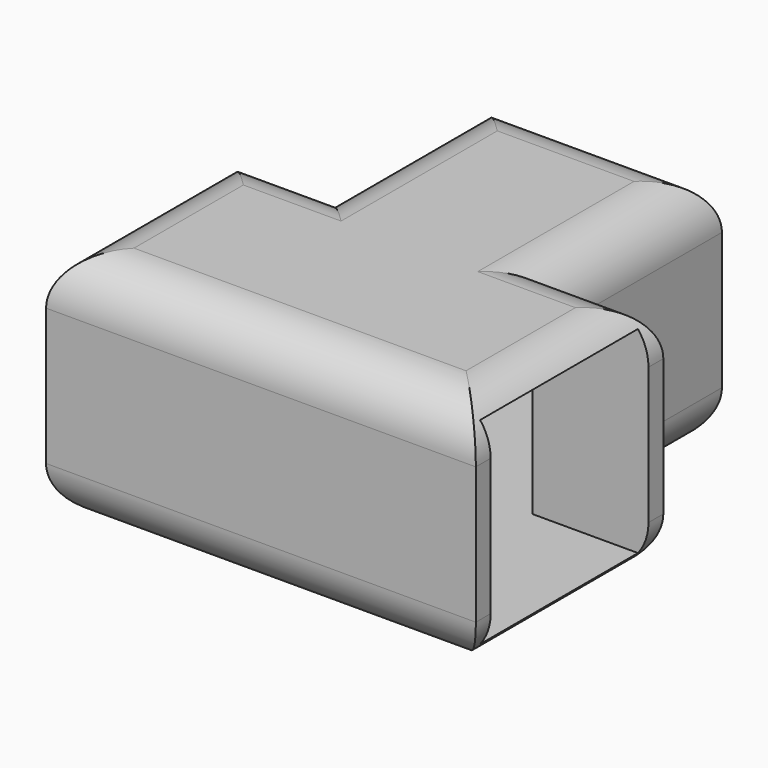
from build123d import *

# Parameters (mm, degrees)
F0_W          = 10
F0_H          = 24
F0_W_2        = 24
F0_H_2        = 20
F1_DEPTH      = 24
F2_T          = -1.9
F3_T1_DEPTH   = 44
F3_T3_DEPTH   = 24
F3_T5_DEPTH   = 10
F3_T7_DEPTH   = 20
F3_T9_DEPTH   = 24
F3_T11_DEPTH  = 10
F3_T17_DEPTH  = 56.5
F3_T21_DEPTH  = 36.5
F3_T28_DEPTH  = 56.5
F3_T32_DEPTH  = 36.5
F3_T39_DEPTH  = 22.5
F3_T43_DEPTH  = 36.5
F3_T50_DEPTH  = 22.5
F3_T54_DEPTH  = 32.5
F3_T61_DEPTH  = 32.5
F3_T65_DEPTH  = 36.5
F3_T72_DEPTH  = 32.5
F3_T76_DEPTH  = 36.5
F3_T83_DEPTH  = 32.5
F3_T87_DEPTH  = 22.5
F3_T94_DEPTH  = 22.5
F3_T98_DEPTH  = 36.5
F3_T105_DEPTH = 56.5
F3_T109_DEPTH = 36.5
F3_T116_DEPTH = 56.5
F3_T120_DEPTH = 36.5
F3_T127_DEPTH = 36.5
F3_T131_DEPTH = 22.5
F3_T138_DEPTH = 22.5
F3_T142_DEPTH = 32.5
F3_T149_DEPTH = 32.5
F3_T153_DEPTH = 36.5
F3_T160_DEPTH = 36.5
F3_T164_DEPTH = 32.5
F3_T171_DEPTH = 32.5
F3_T175_DEPTH = 22.5
F3_T182_DEPTH = 22.5
F3_T186_DEPTH = 36.5


# Not quite as in the source:
# - a fillet or chamfer that OpenCascade refuses, or shapes differently, is made with other operations: its cross-section is extruded or revolved along the edge and cut away or added


with BuildPart() as f1:
    # F0 (on Top) → F1 (new body)
    with BuildSketch(Plane.XY):
        with Locations((-16.1171973497, 12)):
            Rectangle(F0_W, F0_H)
        with Locations((0.8828026503, 12)):
            Rectangle(F0_W_2, F0_H)
        with Locations((17.8828026503, 12)):
            Rectangle(F0_W, F0_H)
        with Locations((0.8828026503, 34)):
            Rectangle(F0_W_2, F0_H_2)
    extrude(amount=F1_DEPTH)

    # F2
    f2_openings = [f1.faces().sort_by_distance(p)[0] for p in [
        (-21.117197, 12, 12),
        (22.882803, 12, 12),
        (0.882803, 44, 12),
    ]]
    offset(amount=F2_T, openings=f2_openings, kind=Kind.INTERSECTION)

    # F3: fillet of radius 5 on 16 edges, made by hand

    # F3_s2 → F3_t1 (cut)
    with BuildSketch(Plane.YZ.offset(-21.1171973497)):
        with BuildLine():
            ThreePointArc((0, 19), (1.4644660941, 22.5355339059), (5, 24))
            Line((5, 24), (5, 24.1))
            Line((5, 24.1), (-0.1, 24.1))
            Line((-0.1, 24.1), (-0.1, 19))
            Line((-0.1, 19), (0, 19))
        make_face()
        with BuildLine():
            ThreePointArc((0, 5), (1.4644660941, 1.4644660941), (5, 0))
            Line((5, 0), (5, -0.1))
            Line((5, -0.1), (-0.1, -0.1))
            Line((-0.1, -0.1), (-0.1, 5))
            Line((-0.1, 5), (0, 5))
        make_face()
    extrude(amount=F3_T1_DEPTH, mode=Mode.SUBTRACT)

    # F3_s4 → F3_t3 (cut)
    with BuildSketch(Plane.XZ.offset(-24)):
        with BuildLine():
            ThreePointArc((17.8828026503, 24), (21.4183365563, 22.5355339059), (22.8828026503, 19))
            Line((22.8828026503, 19), (22.9828026503, 19))
            Line((22.9828026503, 19), (22.9828026503, 24.1))
            Line((22.9828026503, 24.1), (17.8828026503, 24.1))
            Line((17.8828026503, 24.1), (17.8828026503, 24))
        make_face()
        with BuildLine():
            ThreePointArc((-16.1171973497, 24), (-19.6527312556, 22.5355339059), (-21.1171973497, 19))
            Line((-21.1171973497, 19), (-21.2171973497, 19))
            Line((-21.2171973497, 19), (-21.2171973497, 24.1))
            Line((-21.2171973497, 24.1), (-16.1171973497, 24.1))
            Line((-16.1171973497, 24.1), (-16.1171973497, 24))
        make_face()
        with BuildLine():
            ThreePointArc((17.8828026503, 0), (21.4183365563, 1.4644660941), (22.8828026503, 5))
            Line((22.8828026503, 5), (22.9828026503, 5))
            Line((22.9828026503, 5), (22.9828026503, -0.1))
            Line((22.9828026503, -0.1), (17.8828026503, -0.1))
            Line((17.8828026503, -0.1), (17.8828026503, 0))
        make_face()
        with BuildLine():
            ThreePointArc((-16.1171973497, 0), (-19.6527312556, 1.4644660941), (-21.1171973497, 5))
            Line((-21.1171973497, 5), (-21.2171973497, 5))
            Line((-21.2171973497, 5), (-21.2171973497, -0.1))
            Line((-21.2171973497, -0.1), (-16.1171973497, -0.1))
            Line((-16.1171973497, -0.1), (-16.1171973497, 0))
        make_face()
    extrude(amount=F3_T3_DEPTH, mode=Mode.SUBTRACT)

    # F3_s6 → F3_t5 (cut)
    with BuildSketch(Plane.YZ.offset(12.8828026503)):
        with BuildLine():
            ThreePointArc((24, 19), (22.5355339059, 22.5355339059), (19, 24))
            Line((19, 24), (19, 24.1))
            Line((19, 24.1), (24.1, 24.1))
            Line((24.1, 24.1), (24.1, 19))
            Line((24.1, 19), (24, 19))
        make_face()
        with BuildLine():
            ThreePointArc((19, 0), (22.5355339059, 1.4644660941), (24, 5))
            Line((24, 5), (24.1, 5))
            Line((24.1, 5), (24.1, -0.1))
            Line((24.1, -0.1), (19, -0.1))
            Line((19, -0.1), (19, 0))
        make_face()
    extrude(amount=F3_T5_DEPTH, mode=Mode.SUBTRACT)

    # F3_s8 → F3_t7 (cut)
    with BuildSketch(Plane.XZ.offset(-44)):
        with BuildLine():
            ThreePointArc((12.8828026503, 19), (11.4183365563, 22.5355339059), (7.8828026503, 24))
            Line((7.8828026503, 24), (7.8828026503, 24.1))
            Line((7.8828026503, 24.1), (12.9828026503, 24.1))
            Line((12.9828026503, 24.1), (12.9828026503, 19))
            Line((12.9828026503, 19), (12.8828026503, 19))
        make_face()
        with BuildLine():
            ThreePointArc((-11.1171973497, 19), (-9.6527312556, 22.5355339059), (-6.1171973497, 24))
            Line((-6.1171973497, 24), (-6.1171973497, 24.1))
            Line((-6.1171973497, 24.1), (-11.2171973497, 24.1))
            Line((-11.2171973497, 24.1), (-11.2171973497, 19))
            Line((-11.2171973497, 19), (-11.1171973497, 19))
        make_face()
        with BuildLine():
            ThreePointArc((7.8828026503, 0), (11.4183365563, 1.4644660941), (12.8828026503, 5))
            Line((12.8828026503, 5), (12.9828026503, 5))
            Line((12.9828026503, 5), (12.9828026503, -0.1))
            Line((12.9828026503, -0.1), (7.8828026503, -0.1))
            Line((7.8828026503, -0.1), (7.8828026503, 0))
        make_face()
        with BuildLine():
            ThreePointArc((-6.1171973497, 0), (-9.6527312556, 1.4644660941), (-11.1171973497, 5))
            Line((-11.1171973497, 5), (-11.2171973497, 5))
            Line((-11.2171973497, 5), (-11.2171973497, -0.1))
            Line((-11.2171973497, -0.1), (-6.1171973497, -0.1))
            Line((-6.1171973497, -0.1), (-6.1171973497, 0))
        make_face()
    extrude(amount=F3_T7_DEPTH, mode=Mode.SUBTRACT)

    # F3_s10 → F3_t9 (cut)
    with BuildSketch(Plane.YZ.offset(-11.1171973497)):
        with BuildLine():
            ThreePointArc((39, 24), (42.5355339059, 22.5355339059), (44, 19))
            Line((44, 19), (44.1, 19))
            Line((44.1, 19), (44.1, 24.1))
            Line((44.1, 24.1), (39, 24.1))
            Line((39, 24.1), (39, 24))
        make_face()
        with BuildLine():
            ThreePointArc((39, 0), (42.5355339059, 1.4644660941), (44, 5))
            Line((44, 5), (44.1, 5))
            Line((44.1, 5), (44.1, -0.1))
            Line((44.1, -0.1), (39, -0.1))
            Line((39, -0.1), (39, 0))
        make_face()
    extrude(amount=F3_T9_DEPTH, mode=Mode.SUBTRACT)

    # F3_s12 → F3_t11 (cut)
    with BuildSketch(Plane.YZ.offset(-21.1171973497)):
        with BuildLine():
            ThreePointArc((24, 19), (22.5355339059, 22.5355339059), (19, 24))
            Line((19, 24), (19, 24.1))
            Line((19, 24.1), (24.1, 24.1))
            Line((24.1, 24.1), (24.1, 19))
            Line((24.1, 19), (24, 19))
        make_face()
        with BuildLine():
            ThreePointArc((19, 0), (22.5355339059, 1.4644660941), (24, 5))
            Line((24, 5), (24.1, 5))
            Line((24.1, 5), (24.1, -0.1))
            Line((24.1, -0.1), (19, -0.1))
            Line((19, -0.1), (19, 0))
        make_face()
    extrude(amount=F3_T11_DEPTH, mode=Mode.SUBTRACT)


with BuildPart() as f3_tool15:
    # F3_s16 → F3_t17 (new body)
    with BuildSketch(Plane.YZ.offset(-33.6171973497)):
        with BuildLine():
            ThreePointArc((0, 19), (1.4644660941, 22.5355339059), (5, 24))
            Line((5, 24), (5, 24.1))
            Line((5, 24.1), (-0.1, 24.1))
            Line((-0.1, 24.1), (-0.1, 19))
            Line((-0.1, 19), (0, 19))
        make_face()
    extrude(amount=F3_T17_DEPTH)

    split(bisect_by=Plane.YZ.offset(-21.1171973497), keep=Keep.BOTTOM)


with BuildPart() as f3_tool19:
    # F3_s20 → F3_t21 (new body)
    with BuildSketch(Plane.XZ.offset(-24)):
        with BuildLine():
            ThreePointArc((-16.1171973497, 24), (-19.6527312556, 22.5355339059), (-21.1171973497, 19))
            Line((-21.1171973497, 19), (-21.2171973497, 19))
            Line((-21.2171973497, 19), (-21.2171973497, 24.1))
            Line((-21.2171973497, 24.1), (-16.1171973497, 24.1))
            Line((-16.1171973497, 24.1), (-16.1171973497, 24))
        make_face()
    extrude(amount=F3_T21_DEPTH)

    split(bisect_by=Plane.XZ, keep=Keep.TOP)


with BuildPart() as f3_tool15_1:
    add(f3_tool15.part)

    # F3_t23: intersect F3_tool19
    add(f3_tool19.part, mode=Mode.INTERSECT)


with BuildPart() as f1_1:
    add(f1.part)

    # F3_t13: cut F3_tool15
    add(f3_tool15_1.part, mode=Mode.SUBTRACT)


with BuildPart() as f3_tool26:
    # F3_s27 → F3_t28 (new body)
    with BuildSketch(Plane.YZ.offset(-21.1171973497)):
        with BuildLine():
            ThreePointArc((0, 19), (1.4644660941, 22.5355339059), (5, 24))
            Line((5, 24), (5, 24.1))
            Line((5, 24.1), (-0.1, 24.1))
            Line((-0.1, 24.1), (-0.1, 19))
            Line((-0.1, 19), (0, 19))
        make_face()
    extrude(amount=F3_T28_DEPTH)

    split(bisect_by=Plane.YZ.offset(22.8828026503), keep=Keep.TOP)


with BuildPart() as f3_tool30:
    # F3_s31 → F3_t32 (new body)
    with BuildSketch(Plane.XZ.offset(12.5)):
        with BuildLine():
            ThreePointArc((17.8828026503, 24), (21.4183365563, 22.5355339059), (22.8828026503, 19))
            Line((22.8828026503, 19), (22.9828026503, 19))
            Line((22.9828026503, 19), (22.9828026503, 24.1))
            Line((22.9828026503, 24.1), (17.8828026503, 24.1))
            Line((17.8828026503, 24.1), (17.8828026503, 24))
        make_face()
    extrude(amount=-F3_T32_DEPTH)

    split(bisect_by=Plane.XZ, keep=Keep.TOP)


with BuildPart() as f3_tool26_1:
    add(f3_tool26.part)

    # F3_t34: intersect F3_tool30
    add(f3_tool30.part, mode=Mode.INTERSECT)


with BuildPart() as f1_2:
    add(f1_1.part)

    # F3_t24: cut F3_tool26
    add(f3_tool26_1.part, mode=Mode.SUBTRACT)


with BuildPart() as f3_tool37:
    # F3_s38 → F3_t39 (new body)
    with BuildSketch(Plane.YZ.offset(35.3828026503)):
        with BuildLine():
            ThreePointArc((24, 19), (22.5355339059, 22.5355339059), (19, 24))
            Line((19, 24), (19, 24.1))
            Line((19, 24.1), (24.1, 24.1))
            Line((24.1, 24.1), (24.1, 19))
            Line((24.1, 19), (24, 19))
        make_face()
    extrude(amount=-F3_T39_DEPTH)

    split(bisect_by=Plane.YZ.offset(22.8828026503), keep=Keep.TOP)


with BuildPart() as f3_tool41:
    # F3_s42 → F3_t43 (new body)
    with BuildSketch(Plane.XZ):
        with BuildLine():
            ThreePointArc((17.8828026503, 24), (21.4183365563, 22.5355339059), (22.8828026503, 19))
            Line((22.8828026503, 19), (22.9828026503, 19))
            Line((22.9828026503, 19), (22.9828026503, 24.1))
            Line((22.9828026503, 24.1), (17.8828026503, 24.1))
            Line((17.8828026503, 24.1), (17.8828026503, 24))
        make_face()
    extrude(amount=-F3_T43_DEPTH)

    split(bisect_by=Plane.XZ.offset(-24), keep=Keep.BOTTOM)


with BuildPart() as f3_tool37_1:
    add(f3_tool37.part)

    # F3_t45: intersect F3_tool41
    add(f3_tool41.part, mode=Mode.INTERSECT)


with BuildPart() as f1_3:
    add(f1_2.part)

    # F3_t35: cut F3_tool37
    add(f3_tool37_1.part, mode=Mode.SUBTRACT)


with BuildPart() as f3_tool48:
    # F3_s49 → F3_t50 (new body)
    with BuildSketch(Plane.YZ.offset(22.8828026503)):
        with BuildLine():
            ThreePointArc((24, 19), (22.5355339059, 22.5355339059), (19, 24))
            Line((19, 24), (19, 24.1))
            Line((19, 24.1), (24.1, 24.1))
            Line((24.1, 24.1), (24.1, 19))
            Line((24.1, 19), (24, 19))
        make_face()
    extrude(amount=-F3_T50_DEPTH)

    split(bisect_by=Plane.YZ.offset(12.8828026503), keep=Keep.BOTTOM)


with BuildPart() as f3_tool52:
    # F3_s53 → F3_t54 (new body)
    with BuildSketch(Plane.XZ.offset(-11.5)):
        with BuildLine():
            ThreePointArc((12.8828026503, 19), (11.4183365563, 22.5355339059), (7.8828026503, 24))
            Line((7.8828026503, 24), (7.8828026503, 24.1))
            Line((7.8828026503, 24.1), (12.9828026503, 24.1))
            Line((12.9828026503, 24.1), (12.9828026503, 19))
            Line((12.9828026503, 19), (12.8828026503, 19))
        make_face()
    extrude(amount=-F3_T54_DEPTH)

    split(bisect_by=Plane.XZ.offset(-24), keep=Keep.TOP)


with BuildPart() as f3_tool48_1:
    add(f3_tool48.part)

    # F3_t56: intersect F3_tool52
    add(f3_tool52.part, mode=Mode.INTERSECT)


with BuildPart() as f1_4:
    add(f1_3.part)

    # F3_t46: cut F3_tool48
    add(f3_tool48_1.part, mode=Mode.SUBTRACT)


with BuildPart() as f3_tool59:
    # F3_s60 → F3_t61 (new body)
    with BuildSketch(Plane.XZ.offset(-24)):
        with BuildLine():
            ThreePointArc((12.8828026503, 19), (11.4183365563, 22.5355339059), (7.8828026503, 24))
            Line((7.8828026503, 24), (7.8828026503, 24.1))
            Line((7.8828026503, 24.1), (12.9828026503, 24.1))
            Line((12.9828026503, 24.1), (12.9828026503, 19))
            Line((12.9828026503, 19), (12.8828026503, 19))
        make_face()
    extrude(amount=-F3_T61_DEPTH)

    split(bisect_by=Plane.XZ.offset(-44), keep=Keep.BOTTOM)


with BuildPart() as f3_tool63:
    # F3_s64 → F3_t65 (new body)
    with BuildSketch(Plane.YZ.offset(25.3828026503)):
        with BuildLine():
            ThreePointArc((39, 24), (42.5355339059, 22.5355339059), (44, 19))
            Line((44, 19), (44.1, 19))
            Line((44.1, 19), (44.1, 24.1))
            Line((44.1, 24.1), (39, 24.1))
            Line((39, 24.1), (39, 24))
        make_face()
    extrude(amount=-F3_T65_DEPTH)

    split(bisect_by=Plane.YZ.offset(12.8828026503), keep=Keep.TOP)


with BuildPart() as f3_tool59_1:
    add(f3_tool59.part)

    # F3_t67: intersect F3_tool63
    add(f3_tool63.part, mode=Mode.INTERSECT)


with BuildPart() as f1_5:
    add(f1_4.part)

    # F3_t57: cut F3_tool59
    add(f3_tool59_1.part, mode=Mode.SUBTRACT)


with BuildPart() as f3_tool70:
    # F3_s71 → F3_t72 (new body)
    with BuildSketch(Plane.XZ.offset(-56.5)):
        with BuildLine():
            ThreePointArc((-11.1171973497, 19), (-9.6527312556, 22.5355339059), (-6.1171973497, 24))
            Line((-6.1171973497, 24), (-6.1171973497, 24.1))
            Line((-6.1171973497, 24.1), (-11.2171973497, 24.1))
            Line((-11.2171973497, 24.1), (-11.2171973497, 19))
            Line((-11.2171973497, 19), (-11.1171973497, 19))
        make_face()
    extrude(amount=F3_T72_DEPTH)

    split(bisect_by=Plane.XZ.offset(-44), keep=Keep.BOTTOM)


with BuildPart() as f3_tool74:
    # F3_s75 → F3_t76 (new body)
    with BuildSketch(Plane.YZ.offset(12.8828026503)):
        with BuildLine():
            ThreePointArc((39, 24), (42.5355339059, 22.5355339059), (44, 19))
            Line((44, 19), (44.1, 19))
            Line((44.1, 19), (44.1, 24.1))
            Line((44.1, 24.1), (39, 24.1))
            Line((39, 24.1), (39, 24))
        make_face()
    extrude(amount=-F3_T76_DEPTH)

    split(bisect_by=Plane.YZ.offset(-11.1171973497), keep=Keep.BOTTOM)


with BuildPart() as f3_tool70_1:
    add(f3_tool70.part)

    # F3_t78: intersect F3_tool74
    add(f3_tool74.part, mode=Mode.INTERSECT)


with BuildPart() as f1_6:
    add(f1_5.part)

    # F3_t68: cut F3_tool70
    add(f3_tool70_1.part, mode=Mode.SUBTRACT)


with BuildPart() as f3_tool81:
    # F3_s82 → F3_t83 (new body)
    with BuildSketch(Plane.XZ.offset(-44)):
        with BuildLine():
            ThreePointArc((-11.1171973497, 19), (-9.6527312556, 22.5355339059), (-6.1171973497, 24))
            Line((-6.1171973497, 24), (-6.1171973497, 24.1))
            Line((-6.1171973497, 24.1), (-11.2171973497, 24.1))
            Line((-11.2171973497, 24.1), (-11.2171973497, 19))
            Line((-11.2171973497, 19), (-11.1171973497, 19))
        make_face()
    extrude(amount=F3_T83_DEPTH)

    split(bisect_by=Plane.XZ.offset(-24), keep=Keep.TOP)


with BuildPart() as f3_tool85:
    # F3_s86 → F3_t87 (new body)
    with BuildSketch(Plane.YZ.offset(1.3828026503)):
        with BuildLine():
            ThreePointArc((24, 19), (22.5355339059, 22.5355339059), (19, 24))
            Line((19, 24), (19, 24.1))
            Line((19, 24.1), (24.1, 24.1))
            Line((24.1, 24.1), (24.1, 19))
            Line((24.1, 19), (24, 19))
        make_face()
    extrude(amount=-F3_T87_DEPTH)

    split(bisect_by=Plane.YZ.offset(-11.1171973497), keep=Keep.TOP)


with BuildPart() as f3_tool81_1:
    add(f3_tool81.part)

    # F3_t89: intersect F3_tool85
    add(f3_tool85.part, mode=Mode.INTERSECT)


with BuildPart() as f1_7:
    add(f1_6.part)

    # F3_t79: cut F3_tool81
    add(f3_tool81_1.part, mode=Mode.SUBTRACT)


with BuildPart() as f3_tool92:
    # F3_s93 → F3_t94 (new body)
    with BuildSketch(Plane.YZ.offset(-11.1171973497)):
        with BuildLine():
            ThreePointArc((24, 19), (22.5355339059, 22.5355339059), (19, 24))
            Line((19, 24), (19, 24.1))
            Line((19, 24.1), (24.1, 24.1))
            Line((24.1, 24.1), (24.1, 19))
            Line((24.1, 19), (24, 19))
        make_face()
    extrude(amount=-F3_T94_DEPTH)

    split(bisect_by=Plane.YZ.offset(-21.1171973497), keep=Keep.BOTTOM)


with BuildPart() as f3_tool96:
    # F3_s97 → F3_t98 (new body)
    with BuildSketch(Plane.XZ.offset(-36.5)):
        with BuildLine():
            ThreePointArc((-16.1171973497, 24), (-19.6527312556, 22.5355339059), (-21.1171973497, 19))
            Line((-21.1171973497, 19), (-21.2171973497, 19))
            Line((-21.2171973497, 19), (-21.2171973497, 24.1))
            Line((-21.2171973497, 24.1), (-16.1171973497, 24.1))
            Line((-16.1171973497, 24.1), (-16.1171973497, 24))
        make_face()
    extrude(amount=F3_T98_DEPTH)

    split(bisect_by=Plane.XZ.offset(-24), keep=Keep.BOTTOM)


with BuildPart() as f3_tool92_1:
    add(f3_tool92.part)

    # F3_t100: intersect F3_tool96
    add(f3_tool96.part, mode=Mode.INTERSECT)


with BuildPart() as f1_8:
    add(f1_7.part)

    # F3_t90: cut F3_tool92
    add(f3_tool92_1.part, mode=Mode.SUBTRACT)


with BuildPart() as f3_tool103:
    # F3_s104 → F3_t105 (new body)
    with BuildSketch(Plane.YZ.offset(-33.6171973497)):
        with BuildLine():
            ThreePointArc((0, 5), (1.4644660941, 1.4644660941), (5, 0))
            Line((5, 0), (5, -0.1))
            Line((5, -0.1), (-0.1, -0.1))
            Line((-0.1, -0.1), (-0.1, 5))
            Line((-0.1, 5), (0, 5))
        make_face()
    extrude(amount=F3_T105_DEPTH)

    split(bisect_by=Plane.YZ.offset(-21.1171973497), keep=Keep.BOTTOM)


with BuildPart() as f3_tool107:
    # F3_s108 → F3_t109 (new body)
    with BuildSketch(Plane.XZ.offset(-24)):
        with BuildLine():
            ThreePointArc((-16.1171973497, 0), (-19.6527312556, 1.4644660941), (-21.1171973497, 5))
            Line((-21.1171973497, 5), (-21.2171973497, 5))
            Line((-21.2171973497, 5), (-21.2171973497, -0.1))
            Line((-21.2171973497, -0.1), (-16.1171973497, -0.1))
            Line((-16.1171973497, -0.1), (-16.1171973497, 0))
        make_face()
    extrude(amount=F3_T109_DEPTH)

    split(bisect_by=Plane.XZ, keep=Keep.TOP)


with BuildPart() as f3_tool103_1:
    add(f3_tool103.part)

    # F3_t111: intersect F3_tool107
    add(f3_tool107.part, mode=Mode.INTERSECT)


with BuildPart() as f1_9:
    add(f1_8.part)

    # F3_t101: cut F3_tool103
    add(f3_tool103_1.part, mode=Mode.SUBTRACT)


with BuildPart() as f3_tool114:
    # F3_s115 → F3_t116 (new body)
    with BuildSketch(Plane.YZ.offset(-21.1171973497)):
        with BuildLine():
            ThreePointArc((0, 5), (1.4644660941, 1.4644660941), (5, 0))
            Line((5, 0), (5, -0.1))
            Line((5, -0.1), (-0.1, -0.1))
            Line((-0.1, -0.1), (-0.1, 5))
            Line((-0.1, 5), (0, 5))
        make_face()
    extrude(amount=F3_T116_DEPTH)

    split(bisect_by=Plane.YZ.offset(22.8828026503), keep=Keep.TOP)


with BuildPart() as f3_tool118:
    # F3_s119 → F3_t120 (new body)
    with BuildSketch(Plane.XZ.offset(12.5)):
        with BuildLine():
            ThreePointArc((17.8828026503, 0), (21.4183365563, 1.4644660941), (22.8828026503, 5))
            Line((22.8828026503, 5), (22.9828026503, 5))
            Line((22.9828026503, 5), (22.9828026503, -0.1))
            Line((22.9828026503, -0.1), (17.8828026503, -0.1))
            Line((17.8828026503, -0.1), (17.8828026503, 0))
        make_face()
    extrude(amount=-F3_T120_DEPTH)

    split(bisect_by=Plane.XZ, keep=Keep.TOP)


with BuildPart() as f3_tool114_1:
    add(f3_tool114.part)

    # F3_t122: intersect F3_tool118
    add(f3_tool118.part, mode=Mode.INTERSECT)


with BuildPart() as f1_10:
    add(f1_9.part)

    # F3_t112: cut F3_tool114
    add(f3_tool114_1.part, mode=Mode.SUBTRACT)


with BuildPart() as f3_tool125:
    # F3_s126 → F3_t127 (new body)
    with BuildSketch(Plane.XZ):
        with BuildLine():
            ThreePointArc((17.8828026503, 0), (21.4183365563, 1.4644660941), (22.8828026503, 5))
            Line((22.8828026503, 5), (22.9828026503, 5))
            Line((22.9828026503, 5), (22.9828026503, -0.1))
            Line((22.9828026503, -0.1), (17.8828026503, -0.1))
            Line((17.8828026503, -0.1), (17.8828026503, 0))
        make_face()
    extrude(amount=-F3_T127_DEPTH)

    split(bisect_by=Plane.XZ.offset(-24), keep=Keep.BOTTOM)


with BuildPart() as f3_tool129:
    # F3_s130 → F3_t131 (new body)
    with BuildSketch(Plane.YZ.offset(35.3828026503)):
        with BuildLine():
            ThreePointArc((19, 0), (22.5355339059, 1.4644660941), (24, 5))
            Line((24, 5), (24.1, 5))
            Line((24.1, 5), (24.1, -0.1))
            Line((24.1, -0.1), (19, -0.1))
            Line((19, -0.1), (19, 0))
        make_face()
    extrude(amount=-F3_T131_DEPTH)

    split(bisect_by=Plane.YZ.offset(22.8828026503), keep=Keep.TOP)


with BuildPart() as f3_tool125_1:
    add(f3_tool125.part)

    # F3_t133: intersect F3_tool129
    add(f3_tool129.part, mode=Mode.INTERSECT)


with BuildPart() as f1_11:
    add(f1_10.part)

    # F3_t123: cut F3_tool125
    add(f3_tool125_1.part, mode=Mode.SUBTRACT)


with BuildPart() as f3_tool136:
    # F3_s137 → F3_t138 (new body)
    with BuildSketch(Plane.YZ.offset(22.8828026503)):
        with BuildLine():
            ThreePointArc((19, 0), (22.5355339059, 1.4644660941), (24, 5))
            Line((24, 5), (24.1, 5))
            Line((24.1, 5), (24.1, -0.1))
            Line((24.1, -0.1), (19, -0.1))
            Line((19, -0.1), (19, 0))
        make_face()
    extrude(amount=-F3_T138_DEPTH)

    split(bisect_by=Plane.YZ.offset(12.8828026503), keep=Keep.BOTTOM)


with BuildPart() as f3_tool140:
    # F3_s141 → F3_t142 (new body)
    with BuildSketch(Plane.XZ.offset(-11.5)):
        with BuildLine():
            ThreePointArc((7.8828026503, 0), (11.4183365563, 1.4644660941), (12.8828026503, 5))
            Line((12.8828026503, 5), (12.9828026503, 5))
            Line((12.9828026503, 5), (12.9828026503, -0.1))
            Line((12.9828026503, -0.1), (7.8828026503, -0.1))
            Line((7.8828026503, -0.1), (7.8828026503, 0))
        make_face()
    extrude(amount=-F3_T142_DEPTH)

    split(bisect_by=Plane.XZ.offset(-24), keep=Keep.TOP)


with BuildPart() as f3_tool136_1:
    add(f3_tool136.part)

    # F3_t144: intersect F3_tool140
    add(f3_tool140.part, mode=Mode.INTERSECT)


with BuildPart() as f1_12:
    add(f1_11.part)

    # F3_t134: cut F3_tool136
    add(f3_tool136_1.part, mode=Mode.SUBTRACT)


with BuildPart() as f3_tool147:
    # F3_s148 → F3_t149 (new body)
    with BuildSketch(Plane.XZ.offset(-24)):
        with BuildLine():
            ThreePointArc((7.8828026503, 0), (11.4183365563, 1.4644660941), (12.8828026503, 5))
            Line((12.8828026503, 5), (12.9828026503, 5))
            Line((12.9828026503, 5), (12.9828026503, -0.1))
            Line((12.9828026503, -0.1), (7.8828026503, -0.1))
            Line((7.8828026503, -0.1), (7.8828026503, 0))
        make_face()
    extrude(amount=-F3_T149_DEPTH)

    split(bisect_by=Plane.XZ.offset(-44), keep=Keep.BOTTOM)


with BuildPart() as f3_tool151:
    # F3_s152 → F3_t153 (new body)
    with BuildSketch(Plane.YZ.offset(25.3828026503)):
        with BuildLine():
            ThreePointArc((39, 0), (42.5355339059, 1.4644660941), (44, 5))
            Line((44, 5), (44.1, 5))
            Line((44.1, 5), (44.1, -0.1))
            Line((44.1, -0.1), (39, -0.1))
            Line((39, -0.1), (39, 0))
        make_face()
    extrude(amount=-F3_T153_DEPTH)

    split(bisect_by=Plane.YZ.offset(12.8828026503), keep=Keep.TOP)


with BuildPart() as f3_tool147_1:
    add(f3_tool147.part)

    # F3_t155: intersect F3_tool151
    add(f3_tool151.part, mode=Mode.INTERSECT)


with BuildPart() as f1_13:
    add(f1_12.part)

    # F3_t145: cut F3_tool147
    add(f3_tool147_1.part, mode=Mode.SUBTRACT)


with BuildPart() as f3_tool158:
    # F3_s159 → F3_t160 (new body)
    with BuildSketch(Plane.YZ.offset(12.8828026503)):
        with BuildLine():
            ThreePointArc((39, 0), (42.5355339059, 1.4644660941), (44, 5))
            Line((44, 5), (44.1, 5))
            Line((44.1, 5), (44.1, -0.1))
            Line((44.1, -0.1), (39, -0.1))
            Line((39, -0.1), (39, 0))
        make_face()
    extrude(amount=-F3_T160_DEPTH)

    split(bisect_by=Plane.YZ.offset(-11.1171973497), keep=Keep.BOTTOM)


with BuildPart() as f3_tool162:
    # F3_s163 → F3_t164 (new body)
    with BuildSketch(Plane.XZ.offset(-56.5)):
        with BuildLine():
            ThreePointArc((-6.1171973497, 0), (-9.6527312556, 1.4644660941), (-11.1171973497, 5))
            Line((-11.1171973497, 5), (-11.2171973497, 5))
            Line((-11.2171973497, 5), (-11.2171973497, -0.1))
            Line((-11.2171973497, -0.1), (-6.1171973497, -0.1))
            Line((-6.1171973497, -0.1), (-6.1171973497, 0))
        make_face()
    extrude(amount=F3_T164_DEPTH)

    split(bisect_by=Plane.XZ.offset(-44), keep=Keep.BOTTOM)


with BuildPart() as f3_tool158_1:
    add(f3_tool158.part)

    # F3_t166: intersect F3_tool162
    add(f3_tool162.part, mode=Mode.INTERSECT)


with BuildPart() as f1_14:
    add(f1_13.part)

    # F3_t156: cut F3_tool158
    add(f3_tool158_1.part, mode=Mode.SUBTRACT)


with BuildPart() as f3_tool169:
    # F3_s170 → F3_t171 (new body)
    with BuildSketch(Plane.XZ.offset(-44)):
        with BuildLine():
            ThreePointArc((-6.1171973497, 0), (-9.6527312556, 1.4644660941), (-11.1171973497, 5))
            Line((-11.1171973497, 5), (-11.2171973497, 5))
            Line((-11.2171973497, 5), (-11.2171973497, -0.1))
            Line((-11.2171973497, -0.1), (-6.1171973497, -0.1))
            Line((-6.1171973497, -0.1), (-6.1171973497, 0))
        make_face()
    extrude(amount=F3_T171_DEPTH)

    split(bisect_by=Plane.XZ.offset(-24), keep=Keep.TOP)


with BuildPart() as f3_tool173:
    # F3_s174 → F3_t175 (new body)
    with BuildSketch(Plane.YZ.offset(1.3828026503)):
        with BuildLine():
            ThreePointArc((19, 0), (22.5355339059, 1.4644660941), (24, 5))
            Line((24, 5), (24.1, 5))
            Line((24.1, 5), (24.1, -0.1))
            Line((24.1, -0.1), (19, -0.1))
            Line((19, -0.1), (19, 0))
        make_face()
    extrude(amount=-F3_T175_DEPTH)

    split(bisect_by=Plane.YZ.offset(-11.1171973497), keep=Keep.TOP)


with BuildPart() as f3_tool169_1:
    add(f3_tool169.part)

    # F3_t177: intersect F3_tool173
    add(f3_tool173.part, mode=Mode.INTERSECT)


with BuildPart() as f1_15:
    add(f1_14.part)

    # F3_t167: cut F3_tool169
    add(f3_tool169_1.part, mode=Mode.SUBTRACT)


with BuildPart() as f3_tool180:
    # F3_s181 → F3_t182 (new body)
    with BuildSketch(Plane.YZ.offset(-11.1171973497)):
        with BuildLine():
            ThreePointArc((19, 0), (22.5355339059, 1.4644660941), (24, 5))
            Line((24, 5), (24.1, 5))
            Line((24.1, 5), (24.1, -0.1))
            Line((24.1, -0.1), (19, -0.1))
            Line((19, -0.1), (19, 0))
        make_face()
    extrude(amount=-F3_T182_DEPTH)

    split(bisect_by=Plane.YZ.offset(-21.1171973497), keep=Keep.BOTTOM)


with BuildPart() as f3_tool184:
    # F3_s185 → F3_t186 (new body)
    with BuildSketch(Plane.XZ.offset(-36.5)):
        with BuildLine():
            ThreePointArc((-16.1171973497, 0), (-19.6527312556, 1.4644660941), (-21.1171973497, 5))
            Line((-21.1171973497, 5), (-21.2171973497, 5))
            Line((-21.2171973497, 5), (-21.2171973497, -0.1))
            Line((-21.2171973497, -0.1), (-16.1171973497, -0.1))
            Line((-16.1171973497, -0.1), (-16.1171973497, 0))
        make_face()
    extrude(amount=F3_T186_DEPTH)

    split(bisect_by=Plane.XZ.offset(-24), keep=Keep.BOTTOM)


with BuildPart() as f3_tool180_1:
    add(f3_tool180.part)

    # F3_t188: intersect F3_tool184
    add(f3_tool184.part, mode=Mode.INTERSECT)


with BuildPart() as f1_16:
    add(f1_15.part)

    # F3_t178: cut F3_tool180
    add(f3_tool180_1.part, mode=Mode.SUBTRACT)


solid = f1_16.part
